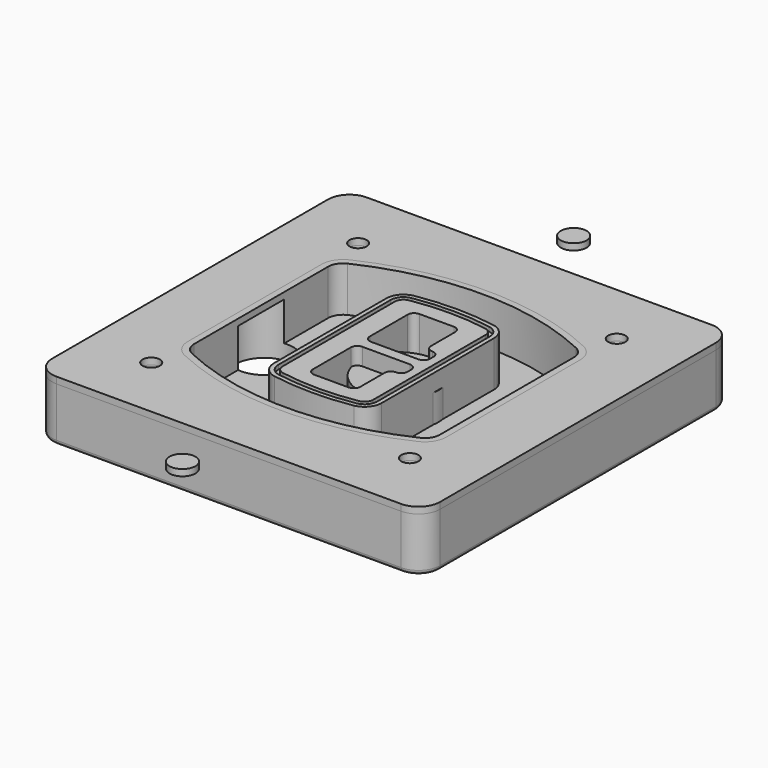
from build123d import *

# Parameters (mm, degrees)
F0_R      = 4
F1_DEPTH  = 25
F2_DEPTH  = 3
F3_DEPTH  = 18
F5_DEPTH  = 21
F6_DEPTH  = 2
F8_DEPTH  = 20
F9_DEPTH  = 16
F10_DEPTH = 25
F7_R      = 6
F7_R_2    = 4
F11_DEPTH = 6
F13_DEPTH = 9
F15_R     = 2
F17_R     = 6
F18_DEPTH = 3
F16_R     = 4


# Not quite as in the source:
# - a feature of the source that left no trace in its solid (it failed there, or was rolled back) is left out
# - a feature names something its author has since deleted; it is built from what else it names


with BuildPart() as f1:
    # F0 (on Top) → F1 (new body)
    with BuildSketch(Plane.XY):
        with BuildLine():
            ThreePointArc((-90, -80), (-87.0710678119, -87.0710678119), (-80, -90))
            Line((-80, -90), (80, -90))
            ThreePointArc((80, -90), (87.0710678119, -87.0710678119), (90, -80))
            Line((90, -80), (90, 80))
            ThreePointArc((90, 80), (87.0710678119, 87.0710678119), (80, 90))
            Line((80, 90), (-80, 90))
            ThreePointArc((-80, 90), (-87.0710678119, 87.0710678119), (-90, 80))
            Line((-90, 80), (-90, -80))
        make_face()
        with Locations((-60, -60)):
            Circle(F0_R, mode=Mode.SUBTRACT)
        with Locations((60, -60)):
            Circle(F0_R, mode=Mode.SUBTRACT)
        with BuildLine():
            ThreePointArc((-64, 38.8308515907), (-61.8195654598, 46.3340424013), (-55.9574468085, 51.5000594398))
            ThreePointArc((-55.9574468085, 51.5000594398), (0, 64), (55.9574468085, 51.5000594398))
            ThreePointArc((55.9574468085, 51.5000594398), (61.8195654598, 46.3340424013), (64, 38.8308515907))
            Line((64, 38.8308515907), (64, -38.8308515907))
            ThreePointArc((64, -38.8308515907), (61.8195654598, -46.3340424013), (55.9574468085, -51.5000594398))
            ThreePointArc((55.9574468085, -51.5000594398), (0, -64), (-55.9574468085, -51.5000594398))
            ThreePointArc((-55.9574468085, -51.5000594398), (-61.8195654598, -46.3340424013), (-64, -38.8308515907))
            Line((-64, -38.8308515907), (-64, 38.8308515907))
        make_face(mode=Mode.SUBTRACT)
        with Locations((-60, 60)):
            Circle(F0_R, mode=Mode.SUBTRACT)
        with Locations((60, 60)):
            Circle(F0_R, mode=Mode.SUBTRACT)
        with BuildLine():
            ThreePointArc((55.9574468085, 51.5000594398), (0, 64), (-55.9574468085, 51.5000594398))
            ThreePointArc((-55.9574468085, 51.5000594398), (-61.8195654598, 46.3340424013), (-64, 38.8308515907))
            Line((-64, 38.8308515907), (-64, -38.8308515907))
            ThreePointArc((-64, -38.8308515907), (-61.8195654598, -46.3340424013), (-55.9574468085, -51.5000594398))
            ThreePointArc((-55.9574468085, -51.5000594398), (0, -64), (55.9574468085, -51.5000594398))
            ThreePointArc((55.9574468085, -51.5000594398), (61.8195654598, -46.3340424013), (64, -38.8308515907))
            Line((64, -38.8308515907), (64, 38.8308515907))
            ThreePointArc((64, 38.8308515907), (61.8195654598, 46.3340424013), (55.9574468085, 51.5000594398))
        make_face()
        with BuildLine():
            Line((-60, -38.8308515907), (-60, 38.8308515907))
            ThreePointArc((-60, 38.8308515907), (-58.442546757, 44.1902735983), (-54.2553191489, 47.8802857686))
            ThreePointArc((-54.2553191489, 47.8802857686), (0, 60), (54.2553191489, 47.8802857686))
            ThreePointArc((54.2553191489, 47.8802857686), (58.442546757, 44.1902735983), (60, 38.8308515907))
            Line((60, 38.8308515907), (60, -38.8308515907))
            ThreePointArc((60, -38.8308515907), (58.442546757, -44.1902735983), (54.2553191489, -47.8802857686))
            ThreePointArc((54.2553191489, -47.8802857686), (0, -60), (-54.2553191489, -47.8802857686))
            ThreePointArc((-54.2553191489, -47.8802857686), (-58.442546757, -44.1902735983), (-60, -38.8308515907))
        make_face(mode=Mode.SUBTRACT)
        with BuildLine():
            ThreePointArc((-54.2553191489, 47.8802857686), (-58.442546757, 44.1902735983), (-60, 38.8308515907))
            Line((-60, 38.8308515907), (-60, -38.8308515907))
            ThreePointArc((-60, -38.8308515907), (-58.442546757, -44.1902735983), (-54.2553191489, -47.8802857686))
            ThreePointArc((-54.2553191489, -47.8802857686), (0, -60), (54.2553191489, -47.8802857686))
            ThreePointArc((54.2553191489, -47.8802857686), (58.442546757, -44.1902735983), (60, -38.8308515907))
            Line((60, -38.8308515907), (60, 38.8308515907))
            ThreePointArc((60, 38.8308515907), (58.442546757, 44.1902735983), (54.2553191489, 47.8802857686))
            ThreePointArc((54.2553191489, 47.8802857686), (0, 60), (-54.2553191489, 47.8802857686))
        make_face()
        with BuildLine():
            ThreePointArc((52.9787234043, 45.1654555152), (55.9097827299, 42.582446996), (57, 38.8308515907))
            Line((57, 38.8308515907), (57, -38.8308515907))
            ThreePointArc((57, -38.8308515907), (55.9097827299, -42.582446996), (52.9787234043, -45.1654555152))
            ThreePointArc((52.9787234043, -45.1654555152), (0, -57), (-52.9787234043, -45.1654555152))
            ThreePointArc((-52.9787234043, -45.1654555152), (-55.9097827299, -42.582446996), (-57, -38.8308515907))
            Line((-57, -38.8308515907), (-57, 38.8308515907))
            ThreePointArc((-57, 38.8308515907), (-55.9097827299, 42.582446996), (-52.9787234043, 45.1654555152))
            ThreePointArc((-52.9787234043, 45.1654555152), (0, 57), (52.9787234043, 45.1654555152))
        make_face(mode=Mode.SUBTRACT)
        with BuildLine():
            Line((57, -38.8308515907), (57, 38.8308515907))
            ThreePointArc((57, 38.8308515907), (55.9097827299, 42.582446996), (52.9787234043, 45.1654555152))
            ThreePointArc((52.9787234043, 45.1654555152), (0, 57), (-52.9787234043, 45.1654555152))
            ThreePointArc((-52.9787234043, 45.1654555152), (-55.9097827299, 42.582446996), (-57, 38.8308515907))
            Line((-57, 38.8308515907), (-57, -38.8308515907))
            ThreePointArc((-57, -38.8308515907), (-55.9097827299, -42.582446996), (-52.9787234043, -45.1654555152))
            ThreePointArc((-52.9787234043, -45.1654555152), (0, -57), (52.9787234043, -45.1654555152))
            ThreePointArc((52.9787234043, -45.1654555152), (55.9097827299, -42.582446996), (57, -38.8308515907))
        make_face()
    extrude(amount=-F1_DEPTH)

    # F0 (on Top) → F2 (join)
    with BuildSketch(Plane.XY):
        with BuildLine():
            ThreePointArc((-54.2553191489, 47.8802857686), (-58.442546757, 44.1902735983), (-60, 38.8308515907))
            Line((-60, 38.8308515907), (-60, -38.8308515907))
            ThreePointArc((-60, -38.8308515907), (-58.442546757, -44.1902735983), (-54.2553191489, -47.8802857686))
            ThreePointArc((-54.2553191489, -47.8802857686), (0, -60), (54.2553191489, -47.8802857686))
            ThreePointArc((54.2553191489, -47.8802857686), (58.442546757, -44.1902735983), (60, -38.8308515907))
            Line((60, -38.8308515907), (60, 38.8308515907))
            ThreePointArc((60, 38.8308515907), (58.442546757, 44.1902735983), (54.2553191489, 47.8802857686))
            ThreePointArc((54.2553191489, 47.8802857686), (0, 60), (-54.2553191489, 47.8802857686))
        make_face()
        with BuildLine():
            ThreePointArc((52.9787234043, 45.1654555152), (55.9097827299, 42.582446996), (57, 38.8308515907))
            Line((57, 38.8308515907), (57, -38.8308515907))
            ThreePointArc((57, -38.8308515907), (55.9097827299, -42.582446996), (52.9787234043, -45.1654555152))
            ThreePointArc((52.9787234043, -45.1654555152), (0, -57), (-52.9787234043, -45.1654555152))
            ThreePointArc((-52.9787234043, -45.1654555152), (-55.9097827299, -42.582446996), (-57, -38.8308515907))
            Line((-57, -38.8308515907), (-57, 38.8308515907))
            ThreePointArc((-57, 38.8308515907), (-55.9097827299, 42.582446996), (-52.9787234043, 45.1654555152))
            ThreePointArc((-52.9787234043, 45.1654555152), (0, 57), (52.9787234043, 45.1654555152))
        make_face(mode=Mode.SUBTRACT)
    extrude(amount=F2_DEPTH)

    # F0 (on Top) → F3 (cut)
    with BuildSketch(Plane.XY):
        with BuildLine():
            Line((57, -38.8308515907), (57, 38.8308515907))
            ThreePointArc((57, 38.8308515907), (55.9097827299, 42.582446996), (52.9787234043, 45.1654555152))
            ThreePointArc((52.9787234043, 45.1654555152), (0, 57), (-52.9787234043, 45.1654555152))
            ThreePointArc((-52.9787234043, 45.1654555152), (-55.9097827299, 42.582446996), (-57, 38.8308515907))
            Line((-57, 38.8308515907), (-57, -38.8308515907))
            ThreePointArc((-57, -38.8308515907), (-55.9097827299, -42.582446996), (-52.9787234043, -45.1654555152))
            ThreePointArc((-52.9787234043, -45.1654555152), (0, -57), (52.9787234043, -45.1654555152))
            ThreePointArc((52.9787234043, -45.1654555152), (55.9097827299, -42.582446996), (57, -38.8308515907))
        make_face()
    extrude(amount=-F3_DEPTH, mode=Mode.SUBTRACT)

    # F4 (on face) → F5 (join, through all)
    with BuildSketch(Plane.XY.offset(3)):
        with BuildLine():
            ThreePointArc((-25, -32.5662280692), (-23.1122504785, -37.7276614059), (-18.3399014778, -40.4532214146))
            ThreePointArc((-18.3399014778, -40.4532214146), (0, -42), (18.3399014778, -40.4532214146))
            ThreePointArc((18.3399014778, -40.4532214146), (23.1122504785, -37.7276614059), (25, -32.5662280692))
            Line((25, -32.5662280692), (25, 32.5662280692))
            ThreePointArc((25, 32.5662280692), (23.1122504785, 37.7276614059), (18.3399014778, 40.4532214146))
            ThreePointArc((18.3399014778, 40.4532214146), (0, 42), (-18.3399014778, 40.4532214146))
            ThreePointArc((-18.3399014778, 40.4532214146), (-23.1122504785, 37.7276614059), (-25, 32.5662280692))
            Line((-25, 32.5662280692), (-25, -32.5662280692))
        make_face()
        with BuildLine():
            ThreePointArc((18.0049261084, 38.4814730782), (21.5841878588, 36.4373030717), (23, 32.5662280692))
            Line((23, 32.5662280692), (23, -32.5662280692))
            ThreePointArc((23, -32.5662280692), (21.5841878588, -36.4373030717), (18.0049261084, -38.4814730782))
            ThreePointArc((18.0049261084, -38.4814730782), (0, -40), (-18.0049261084, -38.4814730782))
            ThreePointArc((-18.0049261084, -38.4814730782), (-21.5841878588, -36.4373030717), (-23, -32.5662280692))
            Line((-23, -32.5662280692), (-23, 32.5662280692))
            ThreePointArc((-23, 32.5662280692), (-21.5841878588, 36.4373030717), (-18.0049261084, 38.4814730782))
            ThreePointArc((-18.0049261084, 38.4814730782), (0, 40), (18.0049261084, 38.4814730782))
        make_face(mode=Mode.SUBTRACT)
        with BuildLine():
            Line((23, -32.5662280692), (23, 32.5662280692))
            ThreePointArc((23, 32.5662280692), (21.5841878588, 36.4373030717), (18.0049261084, 38.4814730782))
            ThreePointArc((18.0049261084, 38.4814730782), (0, 40), (-18.0049261084, 38.4814730782))
            ThreePointArc((-18.0049261084, 38.4814730782), (-21.5841878588, 36.4373030717), (-23, 32.5662280692))
            Line((-23, 32.5662280692), (-23, -32.5662280692))
            ThreePointArc((-23, -32.5662280692), (-21.5841878588, -36.4373030717), (-18.0049261084, -38.4814730782))
            ThreePointArc((-18.0049261084, -38.4814730782), (0, -40), (18.0049261084, -38.4814730782))
            ThreePointArc((18.0049261084, -38.4814730782), (21.5841878588, -36.4373030717), (23, -32.5662280692))
        make_face()
        with BuildLine():
            ThreePointArc((17.6699507389, 36.5097247419), (20.0561252392, 35.1469447375), (21, 32.5662280692))
            Line((21, 32.5662280692), (21, -32.5662280692))
            ThreePointArc((21, -32.5662280692), (20.0561252392, -35.1469447375), (17.6699507389, -36.5097247419))
            ThreePointArc((17.6699507389, -36.5097247419), (0, -38), (-17.6699507389, -36.5097247419))
            ThreePointArc((-17.6699507389, -36.5097247419), (-20.0561252392, -35.1469447375), (-21, -32.5662280692))
            Line((-21, -32.5662280692), (-21, 32.5662280692))
            ThreePointArc((-21, 32.5662280692), (-20.0561252392, 35.1469447375), (-17.6699507389, 36.5097247419))
            ThreePointArc((-17.6699507389, 36.5097247419), (0, 38), (17.6699507389, 36.5097247419))
        make_face(mode=Mode.SUBTRACT)
        with BuildLine():
            Line((21, -32.5662280692), (21, 32.5662280692))
            ThreePointArc((21, 32.5662280692), (20.0561252392, 35.1469447375), (17.6699507389, 36.5097247419))
            ThreePointArc((17.6699507389, 36.5097247419), (0, 38), (-17.6699507389, 36.5097247419))
            ThreePointArc((-17.6699507389, 36.5097247419), (-20.0561252392, 35.1469447375), (-21, 32.5662280692))
            Line((-21, 32.5662280692), (-21, -32.5662280692))
            ThreePointArc((-21, -32.5662280692), (-20.0561252392, -35.1469447375), (-17.6699507389, -36.5097247419))
            ThreePointArc((-17.6699507389, -36.5097247419), (0, -38), (17.6699507389, -36.5097247419))
            ThreePointArc((17.6699507389, -36.5097247419), (20.0561252392, -35.1469447375), (21, -32.5662280692))
        make_face()
        with BuildLine():
            Line((-8, -2.5), (14, -2.5))
            ThreePointArc((14, -2.5), (16.1213203436, -3.3786796564), (17, -5.5))
            Line((17, -5.5), (17, -7.5))
            ThreePointArc((17, -7.5), (16.1213203436, -9.6213203436), (14, -10.5))
            ThreePointArc((14, -10.5), (11.8786796564, -11.3786796564), (11, -13.5))
            Line((11, -13.5), (11, -27.5))
            ThreePointArc((11, -27.5), (10.1213203436, -29.6213203436), (8, -30.5))
            Line((8, -30.5), (-8, -30.5))
            ThreePointArc((-8, -30.5), (-10.1213203436, -29.6213203436), (-11, -27.5))
            Line((-11, -27.5), (-11, -5.5))
            ThreePointArc((-11, -5.5), (-10.1213203436, -3.3786796564), (-8, -2.5))
        make_face(mode=Mode.SUBTRACT)
        with BuildLine():
            ThreePointArc((-8, 2.5), (-10.1213203436, 3.3786796564), (-11, 5.5))
            Line((-11, 5.5), (-11, 27.5))
            ThreePointArc((-11, 27.5), (-10.1213203436, 29.6213203436), (-8, 30.5))
            Line((-8, 30.5), (8, 30.5))
            ThreePointArc((8, 30.5), (10.1213203436, 29.6213203436), (11, 27.5))
            Line((11, 27.5), (11, 13.5))
            ThreePointArc((11, 13.5), (11.8786796564, 11.3786796564), (14, 10.5))
            ThreePointArc((14, 10.5), (16.1213203436, 9.6213203436), (17, 7.5))
            Line((17, 7.5), (17, 5.5))
            ThreePointArc((17, 5.5), (16.1213203436, 3.3786796564), (14, 2.5))
            Line((14, 2.5), (-8, 2.5))
        make_face(mode=Mode.SUBTRACT)
    extrude(amount=-F5_DEPTH)

    # F4 (on face) → F6 (cut)
    with BuildSketch(Plane.XY.offset(3)):
        with BuildLine():
            Line((23, -32.5662280692), (23, 32.5662280692))
            ThreePointArc((23, 32.5662280692), (21.5841878588, 36.4373030717), (18.0049261084, 38.4814730782))
            ThreePointArc((18.0049261084, 38.4814730782), (0, 40), (-18.0049261084, 38.4814730782))
            ThreePointArc((-18.0049261084, 38.4814730782), (-21.5841878588, 36.4373030717), (-23, 32.5662280692))
            Line((-23, 32.5662280692), (-23, -32.5662280692))
            ThreePointArc((-23, -32.5662280692), (-21.5841878588, -36.4373030717), (-18.0049261084, -38.4814730782))
            ThreePointArc((-18.0049261084, -38.4814730782), (0, -40), (18.0049261084, -38.4814730782))
            ThreePointArc((18.0049261084, -38.4814730782), (21.5841878588, -36.4373030717), (23, -32.5662280692))
        make_face()
        with BuildLine():
            ThreePointArc((17.6699507389, 36.5097247419), (20.0561252392, 35.1469447375), (21, 32.5662280692))
            Line((21, 32.5662280692), (21, -32.5662280692))
            ThreePointArc((21, -32.5662280692), (20.0561252392, -35.1469447375), (17.6699507389, -36.5097247419))
            ThreePointArc((17.6699507389, -36.5097247419), (0, -38), (-17.6699507389, -36.5097247419))
            ThreePointArc((-17.6699507389, -36.5097247419), (-20.0561252392, -35.1469447375), (-21, -32.5662280692))
            Line((-21, -32.5662280692), (-21, 32.5662280692))
            ThreePointArc((-21, 32.5662280692), (-20.0561252392, 35.1469447375), (-17.6699507389, 36.5097247419))
            ThreePointArc((-17.6699507389, 36.5097247419), (0, 38), (17.6699507389, 36.5097247419))
        make_face(mode=Mode.SUBTRACT)
    extrude(amount=-F6_DEPTH, mode=Mode.SUBTRACT)

    # F7 (on face) → F8 (join)
    with BuildSketch(Plane(origin=(0, 0, -25), x_dir=(1, 0, 0), z_dir=(0, 0, -1))):
        with BuildLine():
            ThreePointArc((-6.71157564, 0), (6.7567035675, 13.4682792075), (20.224982775, 0))
            Line((20.224982775, 0), (25.224982775, 0))
            ThreePointArc((25.224982775, 0), (6.7567035675, 18.4682792075), (-11.71157564, 0))
            Line((-11.71157564, 0), (-6.71157564, 0))
        make_face()
        with BuildLine():
            Line((-6.71157564, 0), (20.224982775, 0))
            ThreePointArc((20.224982775, 0), (6.7567035675, 13.4682792075), (-6.71157564, 0))
        make_face()
        with BuildLine():
            ThreePointArc((-6.71157564, 0), (6.7567035675, -13.4682792075), (20.224982775, 0))
            Line((20.224982775, 0), (-6.71157564, 0))
        make_face()
        with BuildLine():
            Line((25.224982775, 0), (20.224982775, 0))
            ThreePointArc((20.224982775, 0), (6.7567035675, -13.4682792075), (-6.71157564, 0))
            Line((-6.71157564, 0), (-11.71157564, 0))
            ThreePointArc((-11.71157564, 0), (6.7567035675, -18.4682792075), (25.224982775, 0))
        make_face()
    extrude(amount=-F8_DEPTH)

    # F7 (on face) → F9 (cut)
    with BuildSketch(Plane(origin=(0, 0, -25), x_dir=(1, 0, 0), z_dir=(0, 0, -1))):
        with BuildLine():
            Line((-6.71157564, 0), (20.224982775, 0))
            ThreePointArc((20.224982775, 0), (6.7567035675, 13.4682792075), (-6.71157564, 0))
        make_face()
        with BuildLine():
            ThreePointArc((-6.71157564, 0), (6.7567035675, -13.4682792075), (20.224982775, 0))
            Line((20.224982775, 0), (-6.71157564, 0))
        make_face()
    extrude(amount=-F9_DEPTH, mode=Mode.SUBTRACT)

    # F7 (on face) → F10 (cut)
    with BuildSketch(Plane(origin=(0, 0, -25), x_dir=(1, 0, 0), z_dir=(0, 0, -1))):
        with BuildLine():
            Line((-69.0318229325, 0), (-42.0952645175, 0))
            ThreePointArc((-42.0952645175, 0), (-55.563543725, 13.4682792075), (-69.0318229325, 0))
        make_face()
        with BuildLine():
            ThreePointArc((-69.0318229325, 0), (-55.563543725, -13.4682792075), (-42.0952645175, 0))
            Line((-42.0952645175, 0), (-69.0318229325, 0))
        make_face()
    extrude(amount=-F10_DEPTH, mode=Mode.SUBTRACT)

    # F7 (on face) → F11 (cut)
    with BuildSketch(Plane(origin=(0, 0, -25), x_dir=(1, 0, 0), z_dir=(0, 0, -1))):
        with Locations((60, -60)):
            Circle(F7_R)
        with Locations((60, -60)):
            Circle(F7_R_2, mode=Mode.SUBTRACT)
        with Locations((-60, -60)):
            Circle(F7_R)
        with Locations((-60, -60)):
            Circle(F7_R_2, mode=Mode.SUBTRACT)
        with Locations((-60, 60)):
            Circle(F7_R)
        with Locations((-60, 60)):
            Circle(F7_R_2, mode=Mode.SUBTRACT)
        with Locations((60, 60)):
            Circle(F7_R)
        with Locations((60, 60)):
            Circle(F7_R_2, mode=Mode.SUBTRACT)
    extrude(amount=-F11_DEPTH, mode=Mode.SUBTRACT)

    # F12 (on face) → F13 (cut, through all)
    with BuildSketch(Plane(origin=(0, 0, -9), x_dir=(1, 0, 0), z_dir=(0, 0, -1))):
        with BuildLine():
            ThreePointArc((20.224982775, 0), (20.1663399806, 1.2554664788), (19.9909222755, 2.5))
            Line((19.9909222755, 2.5), (14, 2.5))
            ThreePointArc((14, 2.5), (16.1213203436, 3.3786796564), (17, 5.5))
            Line((17, 5.5), (17, 7.5))
            ThreePointArc((17, 7.5), (16.1213203436, 9.6213203436), (14, 10.5))
            ThreePointArc((14, 10.5), (12.1627255951, 11.1284134507), (11.0951631559, 12.750384826))
            ThreePointArc((11.0951631559, 12.750384826), (11.0476113807, 12.7664660322), (11, 12.7823698976))
            Line((11, 12.7823698976), (11, -12.7823698976))
            ThreePointArc((11, -12.7823698976), (11.0476113807, -12.7664660322), (11.0951631559, -12.750384826))
            ThreePointArc((11.0951631559, -12.750384826), (12.1627255951, -11.1284134507), (14, -10.5))
            ThreePointArc((14, -10.5), (16.1213203436, -9.6213203436), (17, -7.5))
            Line((17, -7.5), (17, -5.5))
            ThreePointArc((17, -5.5), (16.1213203436, -3.3786796564), (14, -2.5))
            Line((14, -2.5), (19.9909222755, -2.5))
            ThreePointArc((19.9909222755, -2.5), (20.1663399806, -1.2554664788), (20.224982775, 0))
        make_face()
    extrude(amount=F13_DEPTH, mode=Mode.SUBTRACT)

    # F15
    f15_edges = [f1.edges().sort_by_distance(p)[0] for p in [
        (0, -90, -25),
        (-87.071068, -87.071068, -25),
        (-90, 0, -25),
        (-87.071068, 87.071068, -25),
        (87.071068, -87.071068, -25),
        (0, 90, -25),
        (90, 0, -25),
        (87.071068, 87.071068, -25),
    ]]
    fillet(f15_edges, radius=F15_R)


with BuildPart() as f18:
    # F17 (on Top) → F18 (new body, through all)
    with BuildSketch(Plane.XY):
        with Locations((-2.7483763946, 113.4528041921)):
            Circle(F17_R)
    extrude(amount=F18_DEPTH)


with BuildPart() as f18b:
    # F17 (on Top) → F18, piece 2 (new body, through all)
    with BuildSketch(Plane.XY):
        with Locations((-2.7483763946, -113.4528041921)):
            Circle(F17_R)
    extrude(amount=F18_DEPTH)


with BuildPart() as f18c:
    # F16 (on face) → F18, piece 3 (new body, through all)
    with BuildSketch(Plane.XY):
        with BuildLine():
            Line((80, 90), (-80, 90))
            ThreePointArc((-80, 90), (-87.0710678119, 87.0710678119), (-90, 80))
            Line((-90, 80), (-90, -80))
            ThreePointArc((-90, -80), (-87.0710678119, -87.0710678119), (-80, -90))
            Line((-80, -90), (80, -90))
            ThreePointArc((80, -90), (87.0710678119, -87.0710678119), (90, -80))
            Line((90, -80), (90, 80))
            ThreePointArc((90, 80), (87.0710678119, 87.0710678119), (80, 90))
        make_face()
        with Locations((-60, -60)):
            Circle(F16_R, mode=Mode.SUBTRACT)
        with Locations((60, -60)):
            Circle(F16_R, mode=Mode.SUBTRACT)
        with Locations((-60, 60)):
            Circle(F16_R, mode=Mode.SUBTRACT)
        with BuildLine():
            Line((-60, -38.8308515907), (-60, 38.8308515907))
            ThreePointArc((-60, 38.8308515907), (-58.442546757, 44.1902735983), (-54.2553191489, 47.8802857686))
            ThreePointArc((-54.2553191489, 47.8802857686), (0, 60), (54.2553191489, 47.8802857686))
            ThreePointArc((54.2553191489, 47.8802857686), (58.442546757, 44.1902735983), (60, 38.8308515907))
            Line((60, 38.8308515907), (60, -38.8308515907))
            ThreePointArc((60, -38.8308515907), (58.442546757, -44.1902735983), (54.2553191489, -47.8802857686))
            ThreePointArc((54.2553191489, -47.8802857686), (0, -60), (-54.2553191489, -47.8802857686))
            ThreePointArc((-54.2553191489, -47.8802857686), (-58.442546757, -44.1902735983), (-60, -38.8308515907))
        make_face(mode=Mode.SUBTRACT)
        with Locations((60, 60)):
            Circle(F16_R, mode=Mode.SUBTRACT)
    extrude(amount=F18_DEPTH)


solid = Compound([f1.part, f18.part, f18b.part, f18c.part])
